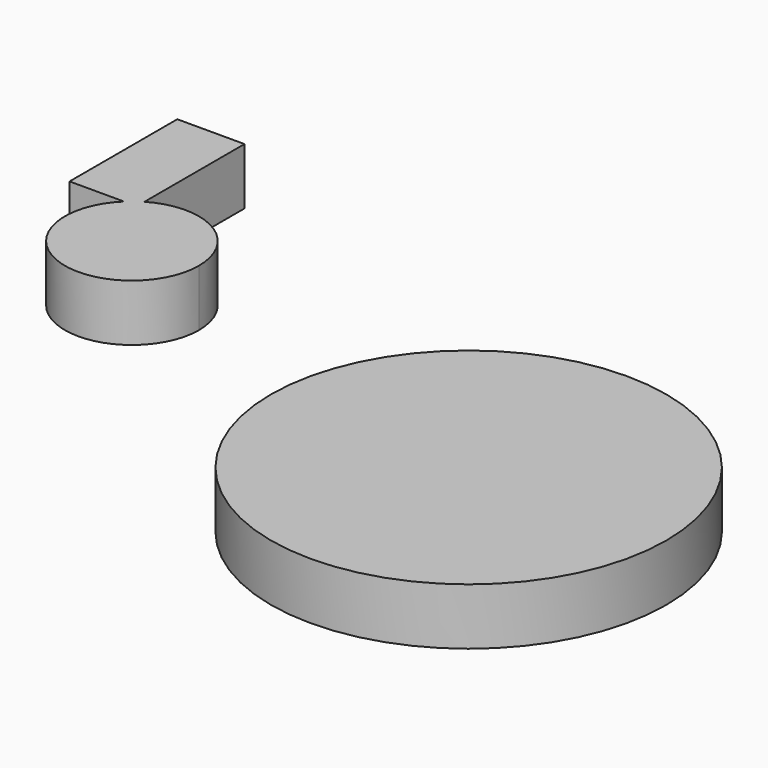
from build123d import *

# Parameters (mm, degrees)
F1_DEPTH = 25.4
F0_R     = 88.5843278601


# Not quite as in the source:
# - a feature names something its author has since deleted; it is built from what else it names


with BuildPart() as f1:
    # F0 (on Top) → F1 (new body)
    with BuildSketch(Plane.XY):
        with BuildLine():
            Line((0, 4.3127644618), (0, 0))
            Line((0, 0), (-5.7035000727, 0))
            ThreePointArc((-5.7035000727, 0), (3.3801290873, -49.2437491092), (45.144380568, -21.6175578535))
            ThreePointArc((45.144380568, -21.6175578535), (30.0768795363, 4.4131774043), (0, 4.3127644618))
        make_face()
        with BuildLine():
            Line((-5.7035000727, 0), (0, 0))
            Line((0, 0), (0, 4.3127644618))
            ThreePointArc((0, 4.3127644618), (-2.9806201388, 2.3268090291), (-5.7035000727, 0))
        make_face()
        with BuildLine():
            Line((-30.1035773009, 0), (-5.7035000727, 0))
            ThreePointArc((-5.7035000727, 0), (-2.9806201388, 2.3268090291), (0, 4.3127644618))
            Line((0, 4.3127644618), (0, 60.3264644742))
            Line((0, 60.3264644742), (-30.1035773009, 60.3264644742))
            Line((-30.1035773009, 60.3264644742), (-30.1035773009, 0))
        make_face()
    extrude(amount=F1_DEPTH)


with BuildPart() as f1b:
    # F0 (on Top) → F1, piece 2 (new body)
    with BuildSketch(Plane.XY):
        with Locations((214.2491787672, -81.9662287831)):
            Circle(F0_R)
    extrude(amount=F1_DEPTH)


solid = Compound([f1.part, f1b.part])
